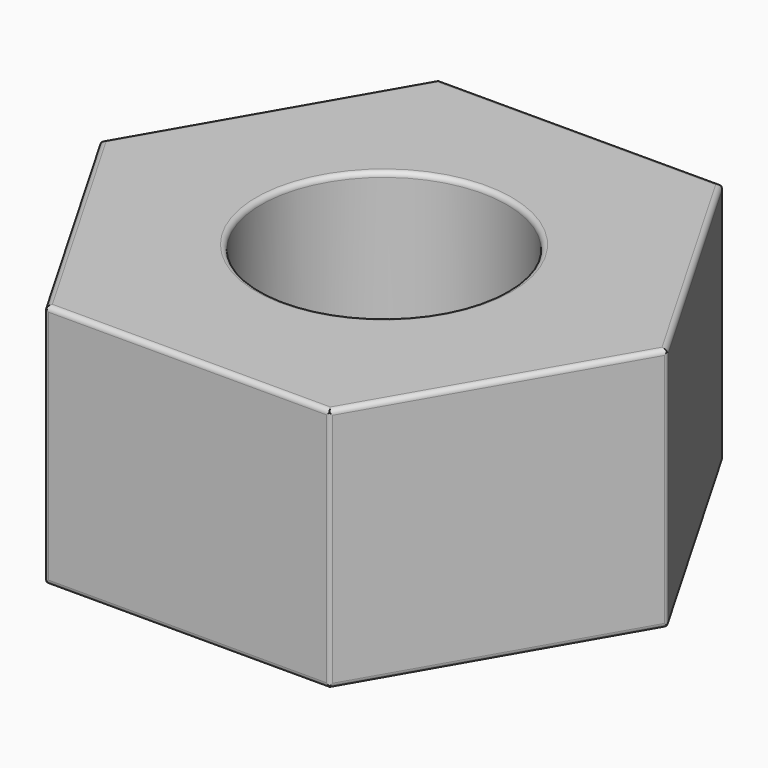
from build123d import *

# Parameters (mm, degrees)
F0_R        = 2.5
F1_DEPTH    = 5
F2_R        = 0.1
F3_T1_DEPTH = 5.0886751346


# Not quite as in the source:
# - a fillet or chamfer that OpenCascade refuses, or shapes differently, is made with other operations: its cross-section is extruded or revolved along the edge and cut away or added


with BuildPart() as f1:
    # F0 (on Top) → F1 (new body)
    with BuildSketch(Plane.XY):
        Polygon((2.8867513459, 5), (-2.8867513459, 5), (-5.7735026919, 0), (-2.8867513459, -5), (2.8867513459, -5), (5.7735026919, 0), align=None)
        Circle(F0_R, mode=Mode.SUBTRACT)
    extrude(amount=F1_DEPTH)

    # F2
    f2_edges = [f1.edges().sort_by_distance(p)[0] for p in [
        (4.330127, 2.5, 0),
        (0, 5, 0),
        (-4.330127, 2.5, 0),
        (-4.330127, -2.5, 0),
        (0, -5, 0),
        (4.330127, -2.5, 0),
        (-2.5, 0, 0),
        (4.330127, 2.5, 5),
        (0, 5, 5),
        (-4.330127, 2.5, 5),
        (-4.330127, -2.5, 5),
        (0, -5, 5),
        (4.330127, -2.5, 5),
        (-2.5, 0, 5),
    ]]
    fillet(f2_edges, radius=F2_R)

    # F3: fillet of radius 0.1 on 18 edges, made by hand

    # F3_s2 → F3_t1 (cut)
    with BuildSketch(Plane.XY.offset(-0.0443375673)):
        with BuildLine():
            ThreePointArc((-2.829016319, 5), (-2.879016319, 4.9866025404), (-2.9156188594, 4.95))
            Line((-2.9156188594, 4.95), (-2.8867513459, 5))
            Line((-2.8867513459, 5), (-2.829016319, 5))
        make_face()
        with BuildLine():
            ThreePointArc((-5.7446351784, 0.05), (-5.7580326381, 0), (-5.7446351784, -0.05))
            Line((-5.7446351784, -0.05), (-5.7735026919, 0))
            Line((-5.7735026919, 0), (-5.7446351784, 0.05))
        make_face()
        with BuildLine():
            ThreePointArc((2.9156188594, 4.95), (2.879016319, 4.9866025404), (2.829016319, 5))
            Line((2.829016319, 5), (2.8867513459, 5))
            Line((2.8867513459, 5), (2.9156188594, 4.95))
        make_face()
        with BuildLine():
            ThreePointArc((5.7446351784, 0.05), (5.7580326381, 0), (5.7446351784, -0.05))
            Line((5.7446351784, -0.05), (5.7735026919, 0))
            Line((5.7735026919, 0), (5.7446351784, 0.05))
        make_face()
        with BuildLine():
            ThreePointArc((-2.829016319, -5), (-2.879016319, -4.9866025404), (-2.9156188594, -4.95))
            Line((-2.9156188594, -4.95), (-2.8867513459, -5))
            Line((-2.8867513459, -5), (-2.829016319, -5))
        make_face()
        with BuildLine():
            ThreePointArc((2.9156188594, -4.95), (2.879016319, -4.9866025404), (2.829016319, -5))
            Line((2.829016319, -5), (2.8867513459, -5))
            Line((2.8867513459, -5), (2.9156188594, -4.95))
        make_face()
    extrude(amount=F3_T1_DEPTH, mode=Mode.SUBTRACT)


solid = f1.part
